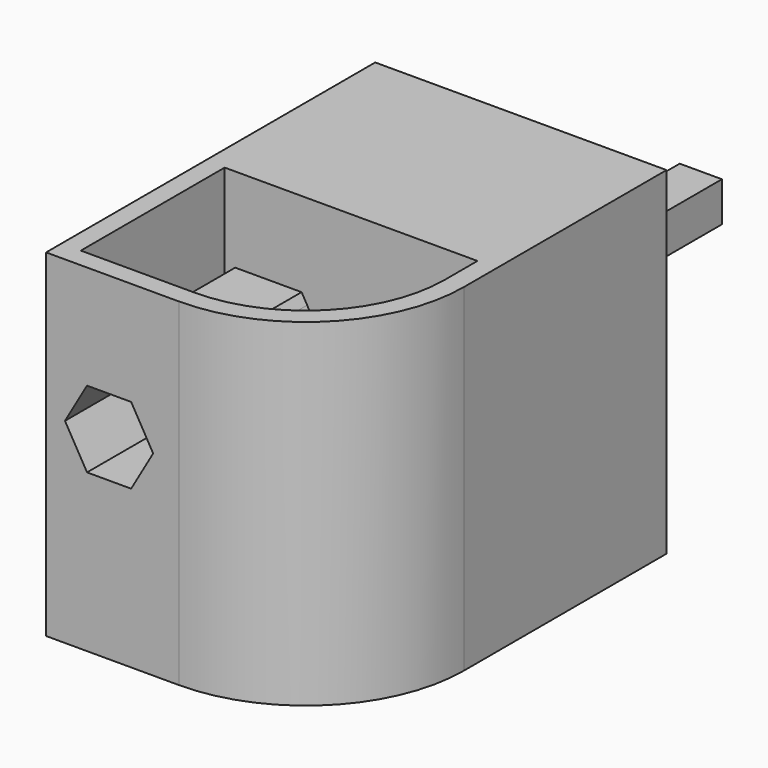
from build123d import *

# Parameters (mm, degrees)
F0_W        = 28.7528
F0_H        = 19.3099416792
F1_DEPTH    = 38.354
F2_DEPTH    = 25.146
F3_R        = 20.8491483247
F5_DEPTH    = 29.972
F6_T        = 2.54
F6_T3_DEPTH = 33.8328
F8_W        = 5.5572818965
F8_H        = 5.2297823131
F9_DEPTH    = 17.78
F9_FACE_W   = 5.5572818965
F9_FACE_H   = 5.2297823131
F7_W        = 38.354
F7_H        = 44.4559416792
F7_R        = 5.5881190885
F10_DEPTH   = 25.4


# Not quite as in the source:
# - a shell that OpenCascade refuses in one call is made with other operations: the cavity is built on its own and cut out


with BuildPart() as f1:
    # F0 (on Right) → F1 (new body)
    with BuildSketch(Plane.YZ):
        with Locations((-45.5179288597, 21.1969297379)):
            Rectangle(F0_W, F0_H)
    extrude(amount=F1_DEPTH)

    # F2 (add): a face of the model
    f2_faces = [f1.faces().sort_by_distance(p)[0] for p in [
        (19.177, -45.5179288597, 30.8519005775),
    ]]
    extrude(f2_faces, amount=F2_DEPTH)

    # F3
    f3_edges = [f1.edges().sort_by_distance(p)[0] for p in [
        (38.354, -59.894329, 33.76993),
    ]]
    fillet(f3_edges, radius=F3_R)

    # F4 (on face) → F5 (cut)
    with BuildSketch(Plane.XZ.offset(59.8943288597)):
        Polygon((5.3893399472, 32.2574861348), (11.1945441877, 32.2574861348), (14.0971463079, 37.2849404812), (11.1945441877, 42.3123948276), (5.3893399472, 42.3123948276), (2.486737827, 37.2849404812), align=None)
    extrude(amount=-F5_DEPTH, mode=Mode.SUBTRACT)

    # F6: shell of thickness 2.54, made by hand


with BuildPart() as f6_core1:
    # F6_t2: copy of F1
    add(f1.part)

    # the walls: a layer under each face that stays
    f6_faces = [f6_core1.faces().sort_by_distance(p)[0] for p in [
        (14.5873763961, -59.8943288597, 48.5885769643),
        (19.177, -45.5179288597, 11.5419588983),
        (32.2474258377, -53.7877546974, 33.7699297379),
        (0, -45.5179288597, 33.7699297379),
        (3.9380388871, -45.5179288597, 39.7986676544),
        (8.2919420674, -45.5179288597, 42.3123948276),
        (12.6458452478, -45.5179288597, 39.7986676544),
        (12.6458452478, -45.5179288597, 34.771213308),
        (8.2919420674, -45.5179288597, 32.2574861348),
        (3.9380388871, -45.5179288597, 34.771213308),
        (38.354, -35.0933546974, 33.7699297379),
        (19.177, -31.1415288597, 33.7699297379),
    ]]
    thicken(f6_faces, amount=-F6_T, mode=Mode.SUBTRACT)

    # F6_s4 → F6_t3 (cut)
    with BuildSketch(Plane.XZ.offset(28.6015288597)):
        Polygon((2.5307319175, 37.2849404812), (0.2870333013, 38.5549404812), (-0.4462015405, 37.2849404812), (0.2870333013, 36.0149404812), align=None)
        Polygon((5.4113369925, 42.2742948276), (3.1896354216, 43.5823948276), (3.9228702635, 44.8523948276), (5.3893399472, 44.8523948276), align=None)
        Polygon((11.1725471424, 42.2742948276), (11.1945441877, 44.8523948276), (12.6610138714, 44.8523948276), (13.3942487133, 43.5823948276), align=None)
        Polygon((14.0531522174, 37.2849404812), (16.2968508335, 38.5549404812), (17.0300856754, 37.2849404812), (16.2968508335, 36.0149404812), align=None)
        Polygon((11.1725471424, 32.2955861348), (13.3942487133, 30.9874861348), (12.6610138714, 29.7174861348), (11.1945441877, 29.7174861348), align=None)
        Polygon((5.4113369925, 32.2955861348), (5.3893399472, 29.7174861348), (3.9228702635, 29.7174861348), (3.1896354216, 30.9874861348), align=None)
    extrude(amount=F6_T3_DEPTH, mode=Mode.SUBTRACT)


with BuildPart() as f1_1:
    add(f1.part)

    # what is left inside the walls is the cavity
    f6_cavity = [f6_core1.part.solids().sort_by_distance(p)[0] for p in [
        (24.722667, -33.706929, 35.03993),
    ]]
    add(f6_cavity, mode=Mode.SUBTRACT)

    # F8 (on face) → F9 (join)
    with BuildSketch(Plane(origin=(0, -31.1415288597, 0), x_dir=(-1, 0, 0), z_dir=(0, 1, 0))):
        with Locations((-28.6376820877, 42.8374167532)):
            Rectangle(F8_W, F8_H)
    extrude(amount=F9_DEPTH)

    # F9_face (on face) + F7 (on face) → F10 (join)
    with BuildSketch(Plane(origin=(28.6376820877, -13.3615288597, 42.8374167532), x_dir=(-1, 0, 0), z_dir=(0, 1, 0))):
        Rectangle(F9_FACE_W, F9_FACE_H)
    with BuildSketch(Plane(origin=(0, -31.1415288597, 0), x_dir=(-1, 0, 0), z_dir=(0, 1, 0))):
        with Locations((-19.177, 33.7699297379)):
            Rectangle(F7_W, F7_H)
        with Locations((-25.0183418393, 30.7178907096)):
            Circle(F7_R, mode=Mode.SUBTRACT)
        Polygon((-5.3893399472, 42.3123948276), (-2.486737827, 37.2849404812), (-5.3893399472, 32.2574861348), (-11.1945441877, 32.2574861348), (-14.0971463079, 37.2849404812), (-11.1945441877, 42.3123948276), align=None, mode=Mode.SUBTRACT)
    extrude(amount=F10_DEPTH)


solid = f1_1.part
